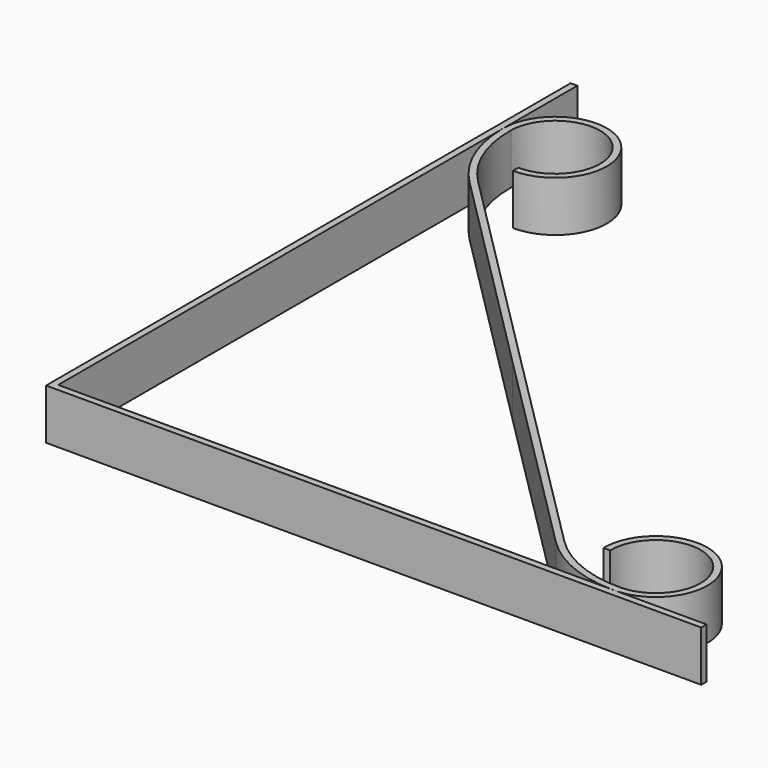
from build123d import *

# Parameters (mm, degrees)
F1_DEPTH = 3.81


# Not quite as in the source:
# - ends of sketch curves that miss each other by under 0.0002 mm in the source are joined


with BuildPart() as f1:
    # F0 (on Top) → F1 (new body)
    with BuildSketch(Plane.XY):
        with BuildLine():
            Line((20.5140408279, -15.1191436985), (-21.2663591647, -15.1191436985))
            Line((-21.2663591647, -15.1191436985), (-21.2358744499, 26.6612451727))
            ThreePointArc((-21.2358744499, 26.6612451727), (-21.2369365638, 26.8078953852), (-21.2356604469, 26.9545438918))
            Line((-21.2356604469, 26.9545438918), (-21.2306322042, 33.8459297569))
            Line((-21.2306322042, 33.8459297569), (-21.7386323148, 33.8459635813))
            Line((-21.7386323148, 33.8459635813), (-21.7747299579, -15.6271436985))
            Line((-21.7747299579, -15.6271436985), (27.6983904911, -15.6271436985))
            Line((27.6983904911, -15.6271436985), (27.6987273246, -15.1191436985))
            Line((27.6987273246, -15.1191436985), (20.8073396251, -15.1191436985))
            ThreePointArc((20.8073396251, -15.1191436985), (20.6606902265, -15.1203128143), (20.5140408279, -15.1191436985))
        make_face()
    extrude(amount=F1_DEPTH)


with BuildPart() as f1b:
    # F0 (on Top) → F1, piece 2 (new body)
    with BuildSketch(Plane.XY):
        with BuildLine():
            Line((-18.5480440044, 20.3022931542), (-2.2025689312, 3.9307418728))
            Line((-2.2025689312, 3.9307418728), (-1.8432276294, 4.2898210799))
            Line((-1.8432276294, 4.2898210799), (-18.1881377204, 20.6608064779))
            Line((-18.1881377204, 20.6608064779), (-18.1885475751, 20.6612169864))
            ThreePointArc((-18.1885475751, 20.6612169864), (-20.0993272211, 23.553656443), (-20.727434667, 26.9628742275))
            ThreePointArc((-20.727434667, 26.9628742275), (-14.8892020702, 29.236140209), (-17.4071495964, 23.4992255697))
            Line((-17.4071495964, 23.4992255697), (-17.4192153155, 22.9913667341))
            ThreePointArc((-17.4192153155, 22.9913667341), (-14.5286368513, 29.5940863142), (-21.2356604469, 26.9545438918))
            Line((-21.2356604469, 26.9545438918), (-21.2358744499, 26.6612451727))
            ThreePointArc((-21.2358744499, 26.6612451727), (-20.5111762537, 23.2200357251), (-18.5480440044, 20.3022931542))
        make_face()
        with BuildLine():
            Line((-1.8432276294, 4.2898210799), (-2.2025689312, 3.9307418728))
            Line((-2.2025689312, 3.9307418728), (14.1570516549, -12.4266742131))
            ThreePointArc((14.1570516549, -12.4266742131), (17.0733610662, -14.3919348459), (20.5140408279, -15.1191436985))
            Line((20.5140408279, -15.1191436985), (20.8073396251, -15.1191436985))
            ThreePointArc((20.8073396251, -15.1191436985), (23.4517750679, -8.414047808), (16.8469481592, -11.2998078844))
            Line((16.8469481592, -11.2998078844), (17.3548156633, -11.2881127234))
            ThreePointArc((17.3548156633, -11.2881127234), (23.0935659746, -8.7743517586), (20.8160725307, -14.6108980778))
            ThreePointArc((20.8160725307, -14.6108980778), (17.4072821975, -13.9803293465), (14.516237695, -12.0674397652))
            ThreePointArc((14.516237695, -12.0674397652), (14.5160325938, -12.0672346847), (14.5158274993, -12.0670295974))
            Line((14.5158274993, -12.0670295974), (-1.8432276294, 4.2898210799))
        make_face()
    extrude(amount=F1_DEPTH)


solid = Compound([f1.part, f1b.part])
